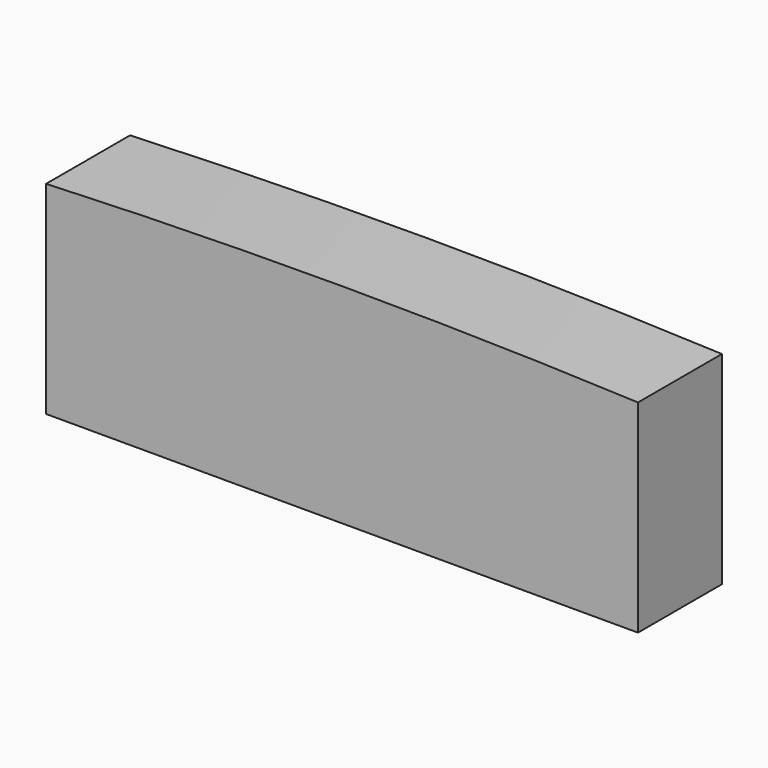
from build123d import *

# Parameters (mm, degrees)
F1_DEPTH = 127


# Not quite as in the source:
# - a feature names something its author has since deleted; it is built from what else it names


with BuildPart() as f1:
    # F0 (on Front) → F1 (new body)
    with BuildSketch(Plane.XZ):
        with BuildLine():
            Line((-358.22686553, 122.6652488112), (-358.22686553, -122.6652488112))
            Line((-358.22686553, -122.6652488112), (358.22686553, -122.6652488112))
            Line((358.22686553, -122.6652488112), (358.22686553, 122.6652488112))
            ThreePointArc((358.22686553, 122.6652488112), (0, 130.0931670637), (-358.22686553, 122.6652488112))
        make_face()
    extrude(amount=F1_DEPTH)


solid = f1.part
